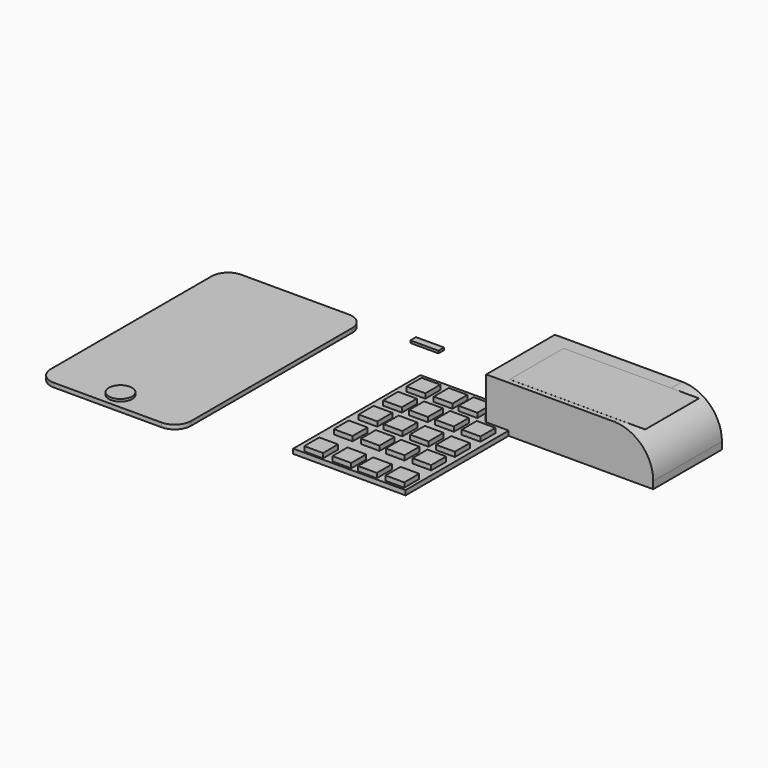
from build123d import *

# Parameters (mm, degrees)
F1_W      = 10.16
F1_H      = 10.16
F2_DEPTH  = 0.508
F4_DEPTH  = 2.286
F0_W      = 60.96
F0_H      = 86.36
F5_DEPTH  = 2.54
F6_R      = 6.35
F7_DEPTH  = 1.27
F8_DEPTH  = 5.08
F9_W      = 15.24
F9_H      = 3.81
F10_DEPTH = 1.27
F11_W     = 90.6102210283
F11_H     = 46.581313014
F12_DEPTH = 25.4
F13_W     = 73.468066752
F13_H     = 36.509571597
F14_DEPTH = 0.0254
F15_R     = 21.4623585695


# Not quite as in the source:
# - a feature names something its author has since deleted; it is built from what else it names


with BuildPart() as f2:
    # F1 (on face) → F2 (new body)
    with BuildSketch(Plane.XY):
        with Locations((7.9427784221, 16.4432588499)):
            Rectangle(F1_W, F1_H)
    extrude(amount=F2_DEPTH)


with BuildPart() as f2b:
    # F1 (on face) → F2, piece 2 (new body)
    with BuildSketch(Plane.XY):
        with Locations((-20.2712472528, 16.4319947362)):
            Rectangle(F1_W, F1_H)
    extrude(amount=F2_DEPTH)


with BuildPart() as f2c:
    # F1 (on face) → F2, piece 3 (new body)
    with BuildSketch(Plane.XY):
        with Locations((-20.4857341331, 32.6637509596)):
            Rectangle(F1_W, F1_H)
    extrude(amount=F2_DEPTH)


with BuildPart() as f2d:
    # F1 (on face) → F2, piece 4 (new body)
    with BuildSketch(Plane.XY):
        with Locations((-5.6699021105, 32.5446701926)):
            Rectangle(F1_W, F1_H)
    extrude(amount=F2_DEPTH)


with BuildPart() as f2e:
    # F1 (on face) → F2, piece 5 (new body)
    with BuildSketch(Plane.XY):
        with Locations((7.8442599307, 32.5446701926)):
            Rectangle(F1_W, F1_H)
    extrude(amount=F2_DEPTH)


with BuildPart() as f2f:
    # F1 (on face) → F2, piece 6 (new body)
    with BuildSketch(Plane.XY):
        with Locations((-20.2712486498, -0.1535746269)):
            Rectangle(F1_W, F1_H)
    extrude(amount=F2_DEPTH)


with BuildPart() as f2g:
    # F1 (on face) → F2, piece 7 (new body)
    with BuildSketch(Plane.XY):
        with Locations((22.4866266045, 16.339353254)):
            Rectangle(F1_W, F1_H)
    extrude(amount=F2_DEPTH)


with BuildPart() as f2h:
    # F1 (on face) → F2, piece 8 (new body)
    with BuildSketch(Plane.XY):
        with Locations((-6.4499458531, -0.4607136361)):
            Rectangle(F1_W, F1_H)
    extrude(amount=F2_DEPTH)


with BuildPart() as f2i:
    # F1 (on face) → F2, piece 9 (new body)
    with BuildSketch(Plane.XY):
        with Locations((8.1514012682, -17.212034637)):
            Rectangle(F1_W, F1_H)
    extrude(amount=F2_DEPTH)


with BuildPart() as f2j:
    # F1 (on face) → F2, piece 10 (new body)
    with BuildSketch(Plane.XY):
        with Locations((22.5869868565, -17.212034637)):
            Rectangle(F1_W, F1_H)
    extrude(amount=F2_DEPTH)


with BuildPart() as f2k:
    # F1 (on face) → F2, piece 11 (new body)
    with BuildSketch(Plane.XY):
        with Locations((9.0728220212, -37.1761438119)):
            Rectangle(F1_W, F1_H)
    extrude(amount=F2_DEPTH)


with BuildPart() as f2l:
    # F1 (on face) → F2, piece 12 (new body)
    with BuildSketch(Plane.XY):
        with Locations((-6.1428144109, 16.4319956675)):
            Rectangle(F1_W, F1_H)
    extrude(amount=F2_DEPTH)


with BuildPart() as f2m:
    # F1 (on face) → F2, piece 13 (new body)
    with BuildSketch(Plane.XY):
        with Locations((22.4212259054, 32.4032818899)):
            Rectangle(F1_W, F1_H)
    extrude(amount=F2_DEPTH)


with BuildPart() as f2n:
    # F1 (on face) → F2, piece 14 (new body)
    with BuildSketch(Plane.XY):
        with Locations((8.1514012682, -0.9336084741)):
            Rectangle(F1_W, F1_H)
    extrude(amount=F2_DEPTH)


with BuildPart() as f2o:
    # F1 (on face) → F2, piece 15 (new body)
    with BuildSketch(Plane.XY):
        with Locations((22.7283667773, -1.3372709826)):
            Rectangle(F1_W, F1_H)
    extrude(amount=F2_DEPTH)


with BuildPart() as f2p:
    # F1 (on face) → F2, piece 16 (new body)
    with BuildSketch(Plane.XY):
        with Locations((-5.6699044389, -16.9048946965)):
            Rectangle(F1_W, F1_H)
    extrude(amount=F2_DEPTH)


with BuildPart() as f2q:
    # F1 (on face) → F2, piece 17 (new body)
    with BuildSketch(Plane.XY):
        with Locations((-5.08, -36.8690010774)):
            Rectangle(F1_W, F1_H)
    extrude(amount=F2_DEPTH)


with BuildPart() as f2r:
    # F1 (on face) → F2, piece 18 (new body)
    with BuildSketch(Plane.XY):
        with Locations((-20.1298664007, -37.1761438119)):
            Rectangle(F1_W, F1_H)
    extrude(amount=F2_DEPTH)


with BuildPart() as f2s:
    # F1 (on face) → F2, piece 19 (new body)
    with BuildSketch(Plane.XY):
        with Locations((-20.1054900271, -17.212034637)):
            Rectangle(F1_W, F1_H)
    extrude(amount=F2_DEPTH)


with BuildPart() as f4:
    # F3 (on Top) → F4 (new body)
    with BuildSketch(Plane.XY):
        with BuildLine():
            Line((-89.2745012665, 68.0546537042), (-147.6945012665, 68.0546537042))
            ThreePointArc((-147.6945012665, 68.0546537042), (-153.9806805512, 65.4508329889), (-156.5845012665, 59.1646537042))
            Line((-156.5845012665, 59.1646537042), (-156.5845012665, -50.0553462958))
            ThreePointArc((-156.5845012665, -50.0553462958), (-153.9806805512, -56.3415255806), (-147.6945012665, -58.9453462958))
            Line((-147.6945012665, -58.9453462958), (-89.2745012665, -58.9453462958))
            ThreePointArc((-89.2745012665, -58.9453462958), (-82.9883219817, -56.3415255806), (-80.3845012665, -50.0553462958))
            Line((-80.3845012665, -50.0553462958), (-80.3845012665, 59.1646537042))
            ThreePointArc((-80.3845012665, 59.1646537042), (-82.9883219817, 65.4508329889), (-89.2745012665, 68.0546537042))
        make_face()
    extrude(amount=F4_DEPTH)

    # F6 (on face) → F7 (join)
    with BuildSketch(Plane.XY.offset(2.286)):
        with Locations((-118.8201233745, -49.9102696776)):
            Circle(F6_R)
    extrude(amount=F7_DEPTH)


with BuildPart() as f5:
    # F0 (on Top) → F5 (new body)
    with BuildSketch(Plane.XY):
        Rectangle(F0_W, F0_H)
    extrude(amount=F5_DEPTH)


with BuildPart() as f8:
    # F1 (on face) → F8 (new body)
    with BuildSketch(Plane.XY):
        with Locations((22.4866266045, 16.339353254)):
            Rectangle(F1_W, F1_H)
    extrude(amount=F8_DEPTH)


with BuildPart() as f8b:
    # F1 (on face) → F8, piece 2 (new body)
    with BuildSketch(Plane.XY):
        with Locations((8.1514012682, -17.212034637)):
            Rectangle(F1_W, F1_H)
    extrude(amount=F8_DEPTH)


with BuildPart() as f8c:
    # F1 (on face) → F8, piece 3 (new body)
    with BuildSketch(Plane.XY):
        with Locations((22.5869868565, -17.212034637)):
            Rectangle(F1_W, F1_H)
    extrude(amount=F8_DEPTH)


with BuildPart() as f8d:
    # F1 (on face) → F8, piece 4 (new body)
    with BuildSketch(Plane.XY):
        with Locations((9.0728220212, -37.1761438119)):
            Rectangle(F1_W, F1_H)
    extrude(amount=F8_DEPTH)


with BuildPart() as f8e:
    # F1 (on face) → F8, piece 5 (new body)
    with BuildSketch(Plane.XY):
        with Locations((-20.4857341331, 32.6637509596)):
            Rectangle(F1_W, F1_H)
    extrude(amount=F8_DEPTH)


with BuildPart() as f8f:
    # F1 (on face) → F8, piece 6 (new body)
    with BuildSketch(Plane.XY):
        with Locations((-6.4499458531, -0.4607136361)):
            Rectangle(F1_W, F1_H)
    extrude(amount=F8_DEPTH)


with BuildPart() as f8g:
    # F1 (on face) → F8, piece 7 (new body)
    with BuildSketch(Plane.XY):
        with Locations((-20.2712486498, -0.1535746269)):
            Rectangle(F1_W, F1_H)
    extrude(amount=F8_DEPTH)


with BuildPart() as f8h:
    # F1 (on face) → F8, piece 8 (new body)
    with BuildSketch(Plane.XY):
        with Locations((-6.1428144109, 16.4319956675)):
            Rectangle(F1_W, F1_H)
    extrude(amount=F8_DEPTH)


with BuildPart() as f8i:
    # F1 (on face) → F8, piece 9 (new body)
    with BuildSketch(Plane.XY):
        with Locations((7.8442599307, 32.5446701926)):
            Rectangle(F1_W, F1_H)
    extrude(amount=F8_DEPTH)


with BuildPart() as f8j:
    # F1 (on face) → F8, piece 10 (new body)
    with BuildSketch(Plane.XY):
        with Locations((-5.6699021105, 32.5446701926)):
            Rectangle(F1_W, F1_H)
    extrude(amount=F8_DEPTH)


with BuildPart() as f8k:
    # F1 (on face) → F8, piece 11 (new body)
    with BuildSketch(Plane.XY):
        with Locations((-20.2712472528, 16.4319947362)):
            Rectangle(F1_W, F1_H)
    extrude(amount=F8_DEPTH)


with BuildPart() as f8l:
    # F1 (on face) → F8, piece 12 (new body)
    with BuildSketch(Plane.XY):
        with Locations((7.9427784221, 16.4432588499)):
            Rectangle(F1_W, F1_H)
    extrude(amount=F8_DEPTH)


with BuildPart() as f8m:
    # F1 (on face) → F8, piece 13 (new body)
    with BuildSketch(Plane.XY):
        with Locations((22.4212259054, 32.4032818899)):
            Rectangle(F1_W, F1_H)
    extrude(amount=F8_DEPTH)


with BuildPart() as f8n:
    # F1 (on face) → F8, piece 14 (new body)
    with BuildSketch(Plane.XY):
        with Locations((8.1514012682, -0.9336084741)):
            Rectangle(F1_W, F1_H)
    extrude(amount=F8_DEPTH)


with BuildPart() as f8o:
    # F1 (on face) → F8, piece 15 (new body)
    with BuildSketch(Plane.XY):
        with Locations((22.7283667773, -1.3372709826)):
            Rectangle(F1_W, F1_H)
    extrude(amount=F8_DEPTH)


with BuildPart() as f8p:
    # F1 (on face) → F8, piece 16 (new body)
    with BuildSketch(Plane.XY):
        with Locations((-20.1054900271, -17.212034637)):
            Rectangle(F1_W, F1_H)
    extrude(amount=F8_DEPTH)


with BuildPart() as f8q:
    # F1 (on face) → F8, piece 17 (new body)
    with BuildSketch(Plane.XY):
        with Locations((-20.1298664007, -37.1761438119)):
            Rectangle(F1_W, F1_H)
    extrude(amount=F8_DEPTH)


with BuildPart() as f8r:
    # F1 (on face) → F8, piece 18 (new body)
    with BuildSketch(Plane.XY):
        with Locations((-5.08, -36.8690010774)):
            Rectangle(F1_W, F1_H)
    extrude(amount=F8_DEPTH)


with BuildPart() as f8s:
    # F1 (on face) → F8, piece 19 (new body)
    with BuildSketch(Plane.XY):
        with Locations((-5.6699044389, -16.9048946965)):
            Rectangle(F1_W, F1_H)
    extrude(amount=F8_DEPTH)


with BuildPart() as f8t:
    # F1 (on face) → F8, piece 20 (new body)
    with BuildSketch(Plane.XY):
        with Locations((23.5751946139, -36.7032434177)):
            Rectangle(F1_W, F1_H)
    extrude(amount=F8_DEPTH)


with BuildPart() as f10:
    # F9 (on Top) → F10 (new body)
    with BuildSketch(Plane.XY):
        with Locations((-47.6863980293, 69.1873268215)):
            Rectangle(F9_W, F9_H)
    extrude(amount=F10_DEPTH)


with BuildPart() as f12:
    # F11 (on Top) → F12 (new body)
    with BuildSketch(Plane.XY):
        with Locations((63.5767802596, 50.0763170421)):
            Rectangle(F11_W, F11_H)
    extrude(amount=F12_DEPTH)

    # F15
    f15_edges = [f12.edges().sort_by_distance(p)[0] for p in [
        (108.881891, 50.076317, 25.4),
    ]]
    fillet(f15_edges, radius=F15_R)


with BuildPart() as f14:
    # F13 (on face) → F14 (new body)
    with BuildSketch(Plane.XY.offset(25.4)):
        with Locations((65.7114870846, 47.642798163)):
            Rectangle(F13_W, F13_H)
    extrude(amount=F14_DEPTH)


solid = Compound([f2.part, f2b.part, f2c.part, f2d.part, f2e.part, f2f.part, f2g.part, f2h.part, f2i.part, f2j.part, f2k.part, f2l.part, f2m.part, f2n.part, f2o.part, f2p.part, f2q.part, f2r.part, f2s.part, f4.part, f5.part, f8.part, f8b.part, f8c.part, f8d.part, f8e.part, f8f.part, f8g.part, f8h.part, f8i.part, f8j.part, f8k.part, f8l.part, f8m.part, f8n.part, f8o.part, f8p.part, f8q.part, f8r.part, f8s.part, f8t.part, f10.part, f12.part, f14.part])
